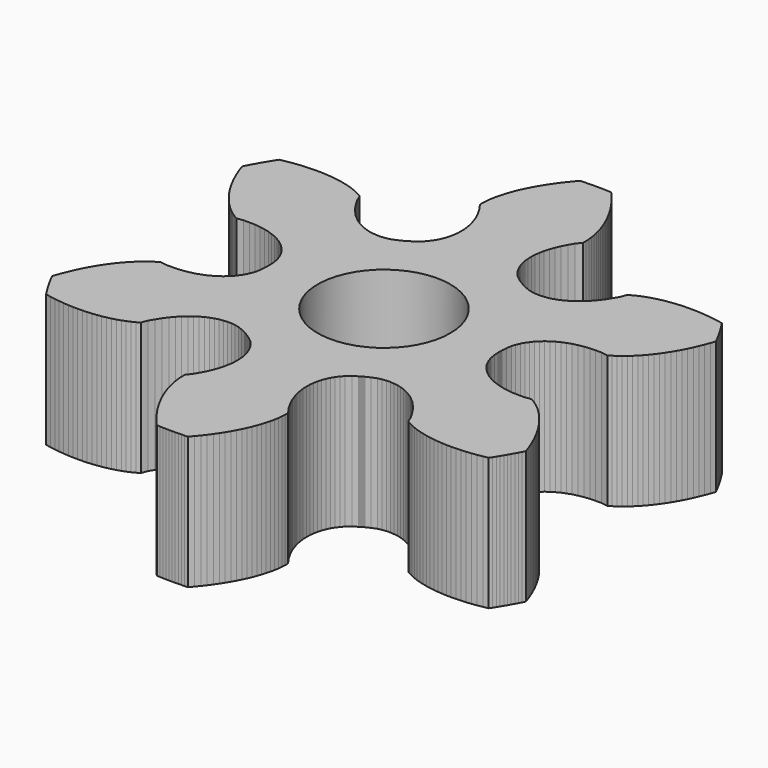
from build123d import *

# Parameters (mm, degrees)
F0_R     = 1.5
F1_DEPTH = 3


# Not quite as in the source:
# - ends of sketch curves that miss each other by under 0.0002 mm in the source are joined


with BuildPart() as f1:
    # F0 (on Top) → F1 (new body)
    with BuildSketch(Plane.XY):
        Polygon((2.624976, -0.011262), (2.625, 0), (2.624976, 0.011262), (2.624903, 0.022524), (2.624783, 0.033786), (2.624613, 0.045047), (2.624396, 0.056308), (2.633586, 0.171193), (2.651847, 0.292005), (2.680751, 0.376262), (2.715885, 0.462448), (2.758346, 0.540199), (2.808501, 0.608479), (2.863261, 0.681367), (2.926303, 0.74242), (2.994733, 0.803776), (3.070282, 0.858596), (3.152728, 0.907843), (3.2411, 0.954754), (3.337429, 0.992187), (3.439087, 1.028728), (3.548992, 1.054145), (3.66447, 1.076865), (3.787388, 1.089881), (3.917258, 1.093874), (4.052295, 1.094222), (4.196763, 1.073649), (4.27202, 1.115769), (4.345558, 1.163911), (4.417501, 1.217224), (4.487882, 1.275207), (4.556695, 1.337523), (4.623912, 1.403922), (4.689487, 1.474211), (4.753369, 1.548229), (4.815497, 1.625845), (4.875808, 1.706941), (4.934234, 1.791414), (4.990706, 1.879168), (5.045153, 1.970116), (5.097502, 2.064175), (5.147679, 2.161265), (5.195612, 2.261311), (5.241226, 2.364236), (5.284447, 2.469969), (5.325202, 2.578436), (5.363417, 2.689565), (5.331429, 2.75243), (5.298703, 2.814914), (5.265246, 2.87701), (5.231061, 2.938708), (5.196152, 3), (5.1605262823, 3.0608777147), (5.1241867469, 3.1213317932), (5.0871385335, 3.1813544051), (5.0493888021, 3.2409379525), (5.0109401151, 3.3000728731), (4.895592078, 3.3225422123), (4.7812794006, 3.341480847), (4.6681014365, 3.356916863), (4.5561587719, 3.3688764802), (4.4455498943, 3.3773882845), (4.3363789879, 3.3824787278), (4.2287470044, 3.384172664), (4.122760226, 3.3824941788), (4.0185270327, 3.3774649922), (3.9161582688, 3.369103092), (3.8157715726, 3.3574202338), (3.7174901449, 3.3424238076), (3.6214476765, 3.3241093727), (3.5277881169, 3.3024642569), (3.4366763961, 3.2774521273), (3.3483026571, 3.2490163212), (3.2628974061, 3.2170560872), (3.1807554937, 3.1814081216), (3.1022942988, 3.1417933455), (3.0281888087, 3.0976788717), (2.9737715494, 2.9622794136), (2.9059516725, 2.8455079412), (2.8375586331, 2.735033722), (2.7648274464, 2.6350916114), (2.6874123493, 2.5464447298), (2.6104480816, 2.4639727078), (2.5279736473, 2.3942047973), (2.4473912184, 2.3294979362), (2.3625791006, 2.2764210392), (2.2787069476, 2.2296442088), (2.193456935, 2.1916268556), (2.1061060803, 2.1630427372), (2.0217116313, 2.1389732637), (1.9312087717, 2.1279937126), (1.8469990571, 2.1186982084), (1.7584342159, 2.1208014038), (1.6662279505, 2.1334674672), (1.578807248, 2.1505643689), (1.465050487, 2.1951558791), (1.3609621584, 2.2446396056), (1.3513183464, 2.2504580331), (1.3416510343, 2.2562357574), (1.3319578562, 2.2619706805), (1.3222411781, 2.2676649003), (1.3125, 2.2733166849), (1.3027348219, 2.2789269003), (1.2929451438, 2.2844946805), (1.2831319657, 2.2900217574), (1.2732946536, 2.2955050331), (1.2634338416, 2.3009476056), (1.168535513, 2.3663488791), (1.073039752, 2.4425693689), (1.0145230495, 2.5097294672), (0.9574507841, 2.5832494038), (0.9113469429, 2.6588972084), (0.8772922283, 2.7364727126), (0.8415493687, 2.8203402637), (0.8201969197, 2.9054627372), (0.801276065, 2.9954028556), (0.7915750524, 3.0882402088), (0.7901488994, 3.1842640392), (0.7937087816, 3.2842519362), (0.8094553527, 3.3863917973), (0.8286389184, 3.4927007078), (0.8615796507, 3.6005897298), (0.8996425536, 3.7119566114), (0.9498293669, 3.824914722), (1.0113063275, 3.9393819412), (1.0785234506, 4.0565014136), (1.1685741913, 4.1713278717), (1.1697257012, 4.2575623455), (1.1648025063, 4.3453191216), (1.1546035939, 4.4342800872), (1.1395793429, 4.5242233212), (1.1200186039, 4.6149751273), (1.0961238831, 4.7063862569), (1.0680393235, 4.7983203727), (1.0358788551, 4.8906528076), (0.9997254274, 4.9832652338), (0.9596497312, 5.076044092), (0.9157069673, 5.1688789922), (0.867945774, 5.2616621788), (0.8164059956, 5.354288664), (0.7611230121, 5.4466537278), (0.7021291057, 5.5386532845), (0.6394532281, 5.6301874802), (0.5731245635, 5.721152863), (0.5031675994, 5.811449847), (0.429609922, 5.9009782123), (0.3524768849, 5.9896378731), (0.2820401979, 5.9933679525), (0.2115644665, 5.9962684051), (0.1410592531, 5.9983417932), (0.0705347177, 5.9995857147), (-2.114e-07, 5.9999996339), (-0.0705347177, 5.9995857147), (-0.1410592531, 5.9983417932), (-0.2115644665, 5.9962684051), (-0.2820401979, 5.9933679525), (-0.3524768849, 5.9896378731), (-0.429609922, 5.9009782123), (-0.5031675994, 5.811449847), (-0.5731245635, 5.721152863), (-0.6394532281, 5.6301874802), (-0.7021291057, 5.5386532845), (-0.7611230121, 5.4466537278), (-0.8164059956, 5.354288664), (-0.867945774, 5.2616621788), (-0.9157069673, 5.1688789922), (-0.9596497312, 5.076044092), (-0.9997254274, 4.9832652338), (-1.0358788551, 4.8906528076), (-1.0680393235, 4.7983203727), (-1.0961238831, 4.7063862569), (-1.1200186039, 4.6149751273), (-1.1395793429, 4.5242233212), (-1.1546035939, 4.4342800872), (-1.1648025063, 4.3453191216), (-1.1697257012, 4.2575623455), (-1.1685741913, 4.1713278717), (-1.0785234506, 4.0565014136), (-1.0113063275, 3.9393819412), (-0.9498293669, 3.824914722), (-0.8996425536, 3.7119566114), (-0.8615796507, 3.6005897298), (-0.8286389184, 3.4927007078), (-0.8094553527, 3.3863917973), (-0.7937087816, 3.2842519362), (-0.7901488994, 3.1842640392), (-0.7915750524, 3.0882402088), (-0.801276065, 2.9954028556), (-0.8201969197, 2.9054627372), (-0.8415493687, 2.8203402637), (-0.8772922283, 2.7364727126), (-0.9113469429, 2.6588972084), (-0.9574507841, 2.5832494038), (-1.0145230495, 2.5097294672), (-1.073039752, 2.4425693689), (-1.168535513, 2.3663488791), (-1.2634338416, 2.3009476056), (-1.2732946536, 2.2955050331), (-1.2831319657, 2.2900217574), (-1.2929451438, 2.2844946805), (-1.3027348219, 2.2789269003), (-1.3125, 2.2733166849), (-1.3222411781, 2.2676649003), (-1.3319578562, 2.2619706805), (-1.3416510343, 2.2562357574), (-1.3513183464, 2.2504580331), (-1.3609621584, 2.2446396056), (-1.465050487, 2.1951558791), (-1.578807248, 2.1505643689), (-1.6662279505, 2.1334674672), (-1.7584342159, 2.1208014038), (-1.8469990571, 2.1186982084), (-1.9312087717, 2.1279937126), (-2.0217116313, 2.1389732637), (-2.1061060803, 2.1630427372), (-2.193456935, 2.1916268556), (-2.2787069476, 2.2296442088), (-2.3625791006, 2.2764210392), (-2.4473912184, 2.3294979362), (-2.5279736473, 2.3942047973), (-2.6104480816, 2.4639727078), (-2.6874123493, 2.5464447298), (-2.7648274464, 2.6350916114), (-2.8375586331, 2.735033722), (-2.9059516725, 2.8455079412), (-2.9737715494, 2.9622794136), (-3.0281888087, 3.0976788717), (-3.1022942988, 3.1417933455), (-3.1807554937, 3.1814081216), (-3.2628974061, 3.2170560872), (-3.3483026571, 3.2490163212), (-3.4366763961, 3.2774521273), (-3.5277881169, 3.3024642569), (-3.6214476765, 3.3241093727), (-3.7174901449, 3.3424238076), (-3.8157715726, 3.3574202338), (-3.9161582688, 3.369103092), (-4.0185270327, 3.3774649922), (-4.122760226, 3.3824941788), (-4.2287470044, 3.384172664), (-4.3363789879, 3.3824787278), (-4.4455498943, 3.3773882845), (-4.5561587719, 3.3688764802), (-4.6681014365, 3.356916863), (-4.7812794006, 3.341480847), (-4.895592078, 3.3225422123), (-5.0109401151, 3.3000728731), (-5.0493888021, 3.2409379525), (-5.0871385335, 3.1813544051), (-5.1241867469, 3.1213317932), (-5.1605262823, 3.0608777147), (-5.1961522114, 2.9999996339), (-5.231061, 2.938708), (-5.265246, 2.87701), (-5.298703, 2.814914), (-5.331429, 2.75243), (-5.363417, 2.689565), (-5.325202, 2.578436), (-5.284447, 2.469969), (-5.241226, 2.364236), (-5.195612, 2.261311), (-5.147679, 2.161265), (-5.097502, 2.064175), (-5.045153, 1.970116), (-4.990706, 1.879168), (-4.934234, 1.791414), (-4.875808, 1.706941), (-4.815497, 1.625845), (-4.753369, 1.548229), (-4.689487, 1.474211), (-4.623912, 1.403922), (-4.556695, 1.337523), (-4.487882, 1.275207), (-4.417501, 1.217224), (-4.345558, 1.163911), (-4.27202, 1.115769), (-4.196763, 1.073649), (-4.052295, 1.094222), (-3.917258, 1.093874), (-3.787388, 1.089881), (-3.66447, 1.076865), (-3.548992, 1.054145), (-3.439087, 1.028728), (-3.337429, 0.992187), (-3.2411, 0.954754), (-3.152728, 0.907843), (-3.070282, 0.858596), (-2.994733, 0.803776), (-2.926303, 0.74242), (-2.863261, 0.681367), (-2.808501, 0.608479), (-2.758346, 0.540199), (-2.715885, 0.462448), (-2.680751, 0.376262), (-2.651847, 0.292005), (-2.633586, 0.171193), (-2.624396, 0.056308), (-2.624613, 0.045047), (-2.624783, 0.033786), (-2.624903, 0.022524), (-2.624976, 0.011262), (-2.625, 0), (-2.624976, -0.011262), (-2.624903, -0.022524), (-2.624783, -0.033786), (-2.624613, -0.045047), (-2.624396, -0.056308), (-2.633586, -0.171193), (-2.651847, -0.292005), (-2.680751, -0.376262), (-2.715885, -0.462448), (-2.758346, -0.540199), (-2.808501, -0.608479), (-2.863261, -0.681367), (-2.926303, -0.74242), (-2.994733, -0.803776), (-3.070282, -0.858596), (-3.152728, -0.907843), (-3.2411, -0.954754), (-3.337429, -0.992187), (-3.439087, -1.028728), (-3.548992, -1.054145), (-3.66447, -1.076865), (-3.787388, -1.089881), (-3.917258, -1.093874), (-4.052295, -1.094222), (-4.196763, -1.073649), (-4.27202, -1.115769), (-4.345558, -1.163911), (-4.417501, -1.217224), (-4.487882, -1.275207), (-4.556695, -1.337523), (-4.623912, -1.403922), (-4.689487, -1.474211), (-4.753369, -1.548229), (-4.815497, -1.625845), (-4.875808, -1.706941), (-4.934234, -1.791414), (-4.990706, -1.879168), (-5.045153, -1.970116), (-5.097502, -2.064175), (-5.147679, -2.161265), (-5.195612, -2.261311), (-5.241226, -2.364236), (-5.284447, -2.469969), (-5.325202, -2.578436), (-5.363417, -2.689565), (-5.331429, -2.75243), (-5.298703, -2.814914), (-5.265246, -2.87701), (-5.231061, -2.938708), (-5.196152, -3), (-5.1605262823, -3.0608777147), (-5.1241867469, -3.1213317932), (-5.0871385335, -3.1813544051), (-5.0493888021, -3.2409379525), (-5.0109401151, -3.3000728731), (-4.895592078, -3.3225422123), (-4.7812794006, -3.341480847), (-4.6681014365, -3.356916863), (-4.5561587719, -3.3688764802), (-4.4455498943, -3.3773882845), (-4.3363789879, -3.3824787278), (-4.2287470044, -3.384172664), (-4.122760226, -3.3824941788), (-4.0185270327, -3.3774649922), (-3.9161582688, -3.369103092), (-3.8157715726, -3.3574202338), (-3.7174901449, -3.3424238076), (-3.6214476765, -3.3241093727), (-3.5277881169, -3.3024642569), (-3.4366763961, -3.2774521273), (-3.3483026571, -3.2490163212), (-3.2628974061, -3.2170560872), (-3.1807554937, -3.1814081216), (-3.1022942988, -3.1417933455), (-3.0281888087, -3.0976788717), (-2.9737715494, -2.9622794136), (-2.9059516725, -2.8455079412), (-2.8375586331, -2.735033722), (-2.7648274464, -2.6350916114), (-2.6874123493, -2.5464447298), (-2.6104480816, -2.4639727078), (-2.5279736473, -2.3942047973), (-2.4473912184, -2.3294979362), (-2.3625791006, -2.2764210392), (-2.2787069476, -2.2296442088), (-2.193456935, -2.1916268556), (-2.1061060803, -2.1630427372), (-2.0217116313, -2.1389732637), (-1.9312087717, -2.1279937126), (-1.8469990571, -2.1186982084), (-1.7584342159, -2.1208014038), (-1.6662279505, -2.1334674672), (-1.578807248, -2.1505643689), (-1.465050487, -2.1951558791), (-1.3609621584, -2.2446396056), (-1.3513183464, -2.2504580331), (-1.3416510343, -2.2562357574), (-1.3319578562, -2.2619706805), (-1.3222411781, -2.2676649003), (-1.3125, -2.2733166849), (-1.3027348219, -2.2789269003), (-1.2929451438, -2.2844946805), (-1.2831319657, -2.2900217574), (-1.2732946536, -2.2955050331), (-1.2634338416, -2.3009476056), (-1.168535513, -2.3663488791), (-1.073039752, -2.4425693689), (-1.0145230495, -2.5097294672), (-0.9574507841, -2.5832494038), (-0.9113469429, -2.6588972084), (-0.8772922283, -2.7364727126), (-0.8415493687, -2.8203402637), (-0.8201969197, -2.9054627372), (-0.801276065, -2.9954028556), (-0.7915750524, -3.0882402088), (-0.7901488994, -3.1842640392), (-0.7937087816, -3.2842519362), (-0.8094553527, -3.3863917973), (-0.8286389184, -3.4927007078), (-0.8615796507, -3.6005897298), (-0.8996425536, -3.7119566114), (-0.9498293669, -3.824914722), (-1.0113063275, -3.9393819412), (-1.0785234506, -4.0565014136), (-1.1685741913, -4.1713278717), (-1.1697257012, -4.2575623455), (-1.1648025063, -4.3453191216), (-1.1546035939, -4.4342800872), (-1.1395793429, -4.5242233212), (-1.1200186039, -4.6149751273), (-1.0961238831, -4.7063862569), (-1.0680393235, -4.7983203727), (-1.0358788551, -4.8906528076), (-0.9997254274, -4.9832652338), (-0.9596497312, -5.076044092), (-0.9157069673, -5.1688789922), (-0.867945774, -5.2616621788), (-0.8164059956, -5.354288664), (-0.7611230121, -5.4466537278), (-0.7021291057, -5.5386532845), (-0.6394532281, -5.6301874802), (-0.5731245635, -5.721152863), (-0.5031675994, -5.811449847), (-0.429609922, -5.9009782123), (-0.3524768849, -5.9896378731), (-0.2820401979, -5.9933679525), (-0.2115644665, -5.9962684051), (-0.1410592531, -5.9983417932), (-0.0705347177, -5.9995857147), (2.114e-07, -5.9999996339), (0.0705347177, -5.9995857147), (0.1410592531, -5.9983417932), (0.2115644665, -5.9962684051), (0.2820401979, -5.9933679525), (0.3524768849, -5.9896378731), (0.429609922, -5.9009782123), (0.5031675994, -5.811449847), (0.5731245635, -5.721152863), (0.6394532281, -5.6301874802), (0.7021291057, -5.5386532845), (0.7611230121, -5.4466537278), (0.8164059956, -5.354288664), (0.867945774, -5.2616621788), (0.9157069673, -5.1688789922), (0.9596497312, -5.076044092), (0.9997254274, -4.9832652338), (1.0358788551, -4.8906528076), (1.0680393235, -4.7983203727), (1.0961238831, -4.7063862569), (1.1200186039, -4.6149751273), (1.1395793429, -4.5242233212), (1.1546035939, -4.4342800872), (1.1648025063, -4.3453191216), (1.1697257012, -4.2575623455), (1.1685741913, -4.1713278717), (1.0785234506, -4.0565014136), (1.0113063275, -3.9393819412), (0.9498293669, -3.824914722), (0.8996425536, -3.7119566114), (0.8615796507, -3.6005897298), (0.8286389184, -3.4927007078), (0.8094553527, -3.3863917973), (0.7937087816, -3.2842519362), (0.7901488994, -3.1842640392), (0.7915750524, -3.0882402088), (0.801276065, -2.9954028556), (0.8201969197, -2.9054627372), (0.8415493687, -2.8203402637), (0.8772922283, -2.7364727126), (0.9113469429, -2.6588972084), (0.9574507841, -2.5832494038), (1.0145230495, -2.5097294672), (1.073039752, -2.4425693689), (1.168535513, -2.3663488791), (1.2634338416, -2.3009476056), (1.2732946536, -2.2955050331), (1.2831319657, -2.2900217574), (1.2929451438, -2.2844946805), (1.3027348219, -2.2789269003), (1.3125, -2.2733166849), (1.3222411781, -2.2676649003), (1.3319578562, -2.2619706805), (1.3416510343, -2.2562357574), (1.3513183464, -2.2504580331), (1.3609621584, -2.2446396056), (1.465050487, -2.1951558791), (1.578807248, -2.1505643689), (1.6662279505, -2.1334674672), (1.7584342159, -2.1208014038), (1.8469990571, -2.1186982084), (1.9312087717, -2.1279937126), (2.0217116313, -2.1389732637), (2.1061060803, -2.1630427372), (2.193456935, -2.1916268556), (2.2787069476, -2.2296442088), (2.3625791006, -2.2764210392), (2.4473912184, -2.3294979362), (2.5279736473, -2.3942047973), (2.6104480816, -2.4639727078), (2.6874123493, -2.5464447298), (2.7648274464, -2.6350916114), (2.8375586331, -2.735033722), (2.9059516725, -2.8455079412), (2.9737715494, -2.9622794136), (3.0281888087, -3.0976788717), (3.1022942988, -3.1417933455), (3.1807554937, -3.1814081216), (3.2628974061, -3.2170560872), (3.3483026571, -3.2490163212), (3.4366763961, -3.2774521273), (3.5277881169, -3.3024642569), (3.6214476765, -3.3241093727), (3.7174901449, -3.3424238076), (3.8157715726, -3.3574202338), (3.9161582688, -3.369103092), (4.0185270327, -3.3774649922), (4.122760226, -3.3824941788), (4.2287470044, -3.384172664), (4.3363789879, -3.3824787278), (4.4455498943, -3.3773882845), (4.5561587719, -3.3688764802), (4.6681014365, -3.356916863), (4.7812794006, -3.341480847), (4.895592078, -3.3225422123), (5.0109401151, -3.3000728731), (5.0493888021, -3.2409379525), (5.0871385335, -3.1813544051), (5.1241867469, -3.1213317932), (5.1605262823, -3.0608777147), (5.1961522114, -2.9999996339), (5.231061, -2.938708), (5.265246, -2.87701), (5.298703, -2.814914), (5.331429, -2.75243), (5.363417, -2.689565), (5.325202, -2.578436), (5.284447, -2.469969), (5.241226, -2.364236), (5.195612, -2.261311), (5.147679, -2.161265), (5.097502, -2.064175), (5.045153, -1.970116), (4.990706, -1.879168), (4.934234, -1.791414), (4.875808, -1.706941), (4.815497, -1.625845), (4.753369, -1.548229), (4.689487, -1.474211), (4.623912, -1.403922), (4.556695, -1.337523), (4.487882, -1.275207), (4.417501, -1.217224), (4.345558, -1.163911), (4.27202, -1.115769), (4.196763, -1.073649), (4.052295, -1.094222), (3.917258, -1.093874), (3.787388, -1.089881), (3.66447, -1.076865), (3.548992, -1.054145), (3.439087, -1.028728), (3.337429, -0.992187), (3.2411, -0.954754), (3.152728, -0.907843), (3.070282, -0.858596), (2.994733, -0.803776), (2.926303, -0.74242), (2.863261, -0.681367), (2.808501, -0.608479), (2.758346, -0.540199), (2.715885, -0.462448), (2.680751, -0.376262), (2.651847, -0.292005), (2.633586, -0.171193), (2.624396, -0.056308), (2.624613, -0.045047), (2.624783, -0.033786), (2.624903, -0.022524), align=None)
        Circle(F0_R, mode=Mode.SUBTRACT)
    extrude(amount=F1_DEPTH)


solid = f1.part
